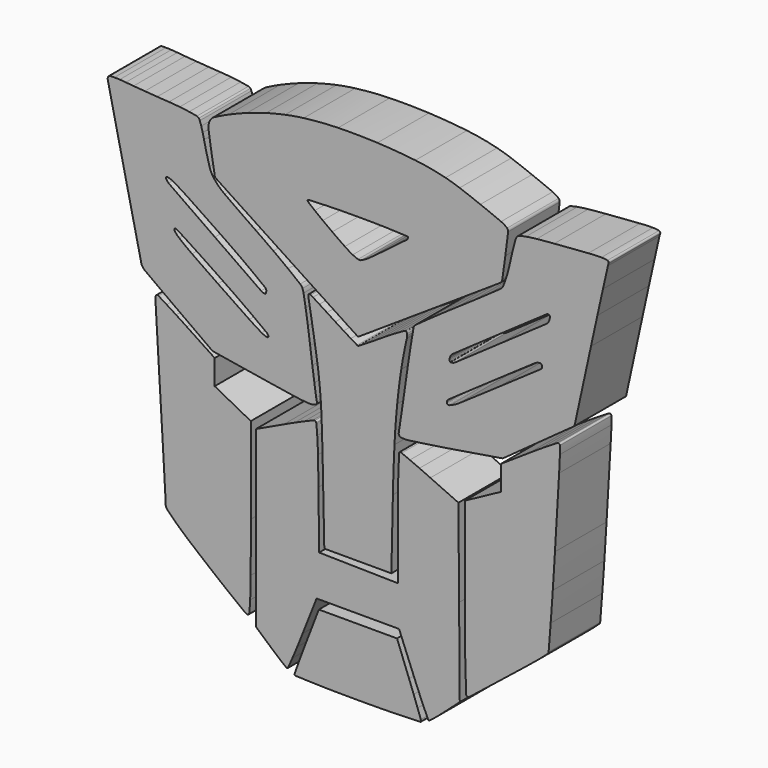
from build123d import *

# Parameters (mm, degrees)
F1_DEPTH = 25


# Not quite as in the source:
# - ends of sketch curves that miss each other by under 0.0002 mm in the source are joined


with BuildPart() as f1:
    # F0 (on Front) → F1 (new body)
    with BuildSketch(Plane.XZ):
        with BuildLine():
            ThreePointArc((-7.7871389968, 96.4009488717), (-14.4802858445, 96.0659455326), (-21.1477259866, 95.3909018942))
            ThreePointArc((-21.1477259866, 95.3909018942), (-24.7777244631, 94.8564824054), (-28.3836838991, 94.1785815164))
            ThreePointArc((-28.3836838991, 94.1785815164), (-32.0904730243, 93.3361025196), (-35.7648669134, 92.3619946955))
            ThreePointArc((-35.7648669134, 92.3619946955), (-39.4624856609, 91.2403059302), (-43.1184530528, 89.9895171458))
            ThreePointArc((-43.1184530528, 89.9895171458), (-46.7206384931, 88.6136238863), (-50.2719786883, 87.1113572979))
            ThreePointArc((-50.2719786883, 87.1113572979), (-53.1174557084, 85.7851246094), (-55.9125031708, 84.3556693195))
            ThreePointArc((-55.9125031708, 84.3556693195), (-56.9599216153, 83.5327385231), (-57.6618821388, 82.4006820555))
            ThreePointArc((-57.6618821388, 82.4006820555), (-58.0273005227, 80.978523326), (-58.0188121091, 79.5101931205))
            ThreePointArc((-58.0188121091, 79.5101931205), (-57.4050586657, 75.2351533659), (-56.7215456466, 70.9707110596))
            Line((-56.7215456466, 70.9707110596), (-55.545967, 64.001086))
            Line((-55.545967, 64.001086), (-30.461838, 47.51707))
            ThreePointArc((-30.461838, 47.51707), (-25.5599805849, 44.2963588564), (-20.6576271192, 41.0764028185))
            ThreePointArc((-20.6576271192, 41.0764028185), (-16.3105522589, 38.2223324949), (-11.9628498638, 35.3692182077))
            ThreePointArc((-11.9628498638, 35.3692182077), (-8.2807722481, 32.9538008658), (-4.5984092513, 30.5388186167))
            ThreePointArc((-4.5984092513, 30.5388186167), (-3.6557973546, 29.9230173812), (-2.7110817564, 29.3104483771))
            Line((-2.7110817564, 29.3104483771), (-0.044454, 27.587842))
            Line((-0.044454, 27.587842), (27.40391, 45.662816))
            ThreePointArc((27.40391, 45.662816), (32.6768790001, 49.136531609), (37.9485342795, 52.6122405762))
            ThreePointArc((37.9485342795, 52.6122405762), (42.4121029737, 55.5583452338), (46.8738502017, 58.5072076951))
            ThreePointArc((46.8738502017, 58.5072076951), (50.8820698473, 61.1582365066), (54.8901678715, 63.8094491942))
            ThreePointArc((54.8901678715, 63.8094491942), (55.0192170204, 63.9027750955), (55.1400437901, 64.0065262248))
            ThreePointArc((55.1400437901, 64.0065262248), (55.6271868144, 64.6463564976), (55.8748182743, 65.4114511053))
            ThreePointArc((55.8748182743, 65.4114511053), (56.4715267421, 69.6147694006), (57.0417758288, 73.8217590227))
            ThreePointArc((57.0417758288, 73.8217590227), (57.596923666, 78.0974834015), (58.1309676384, 82.3758949219))
            ThreePointArc((58.1309676384, 82.3758949219), (58.0590093517, 82.9769076903), (57.7167750279, 83.4761770312))
            ThreePointArc((57.7167750279, 83.4761770312), (56.6161151389, 84.3050714361), (55.392932935, 84.939376844))
            ThreePointArc((55.392932935, 84.939376844), (51.3880107464, 86.5869045709), (47.3681719583, 88.1976948946))
            ThreePointArc((47.3681719583, 88.1976948946), (43.3587549264, 89.7477962193), (39.3261631957, 91.2365685427))
            ThreePointArc((39.3261631957, 91.2365685427), (36.6097303702, 92.1414723377), (33.8522739854, 92.9123759426))
            ThreePointArc((33.8522739854, 92.9123759426), (28.0367501, 94.1819202218), (22.1498009897, 95.0627669114))
            ThreePointArc((22.1498009897, 95.0627669114), (14.802388714, 95.7832710166), (7.4341970002, 96.2451630052))
            ThreePointArc((7.4341970002, 96.2451630052), (-0.1751155832, 96.4554892907), (-7.7871389968, 96.4009488717))
        make_face()
        with BuildLine():
            ThreePointArc((19.0402640372, 68.0878828396), (19.2429014899, 67.9932442976), (19.3193110957, 67.7830539958))
            ThreePointArc((19.3193110957, 67.7830539958), (19.1813400447, 67.2695037039), (18.8389564856, 66.8626336728))
            ThreePointArc((18.8389564856, 66.8626336728), (15.1159629469, 64.0249741693), (11.384749851, 61.1981311973))
            ThreePointArc((11.384749851, 61.1981311973), (7.9259756693, 58.6105934074), (4.4434357694, 56.0551313173))
            ThreePointArc((4.4434357694, 56.0551313173), (2.9054012774, 55.0379035263), (1.2837569665, 54.1600810691))
            ThreePointArc((1.2837569665, 54.1600810691), (0.6198402223, 53.9798990752), (-0.0640028179, 54.0547965969))
            ThreePointArc((-0.0640028179, 54.0547965969), (-1.1212634849, 54.4332391828), (-2.1377660104, 54.9104619803))
            ThreePointArc((-2.1377660104, 54.9104619803), (-3.6865885064, 55.7856963811), (-5.184320766, 56.7457403437))
            ThreePointArc((-5.184320766, 56.7457403437), (-7.6332065318, 58.4369597951), (-10.059751525, 60.1600802708))
            ThreePointArc((-10.059751525, 60.1600802708), (-11.896375827, 61.4957166855), (-13.720253444, 62.8487074074))
            ThreePointArc((-13.720253444, 62.8487074074), (-15.2728438218, 64.0300656839), (-16.8076561206, 65.2344308486))
            ThreePointArc((-16.8076561206, 65.2344308486), (-18.106988474, 66.2756164446), (-19.400562618, 67.3239474687))
            ThreePointArc((-19.400562618, 67.3239474687), (-19.5636563725, 67.5288505749), (-19.6266290148, 67.7830539996))
            ThreePointArc((-19.6266290148, 67.7830539996), (-19.5472806273, 67.9935196361), (-19.3431069986, 68.0878869692))
            ThreePointArc((-19.3431069986, 68.0878869692), (-16.6284187312, 68.2042556562), (-13.9134039882, 68.3127406931))
            ThreePointArc((-13.9134039882, 68.3127406931), (-10.7689410735, 68.4148692664), (-7.6234769951, 68.4791576626))
            ThreePointArc((-7.6234769951, 68.4791576626), (-3.8856986475, 68.5195810383), (-0.147726, 68.5330539999))
            ThreePointArc((-0.147726, 68.5330539999), (3.5898426403, 68.5195815863), (7.327217, 68.4791620031))
            ThreePointArc((7.327217, 68.4791620031), (10.471342585, 68.4148820808), (13.6144659873, 68.3127406712))
            ThreePointArc((13.6144659873, 68.3127406712), (16.3275287109, 68.204261809), (19.0402640372, 68.0878828396))
        make_face(mode=Mode.SUBTRACT)
    extrude(amount=F1_DEPTH)


with BuildPart() as f1b:
    # F0 (on Front) → F1, piece 2 (new body)
    with BuildSketch(Plane.XZ):
        with BuildLine():
            ThreePointArc((-96.2537729873, 85.3507327118), (-96.5128646217, 85.2890918282), (-96.7307979178, 85.1360129205))
            ThreePointArc((-96.7307979178, 85.1360129205), (-97.0917755206, 84.5089297705), (-97.112631726, 83.7856710607))
            ThreePointArc((-97.112631726, 83.7856710607), (-93.8621854047, 69.1270025934), (-90.6031200374, 54.4702479917))
            ThreePointArc((-90.6031200374, 54.4702479917), (-87.3658251329, 39.9600151765), (-84.1164584372, 25.4524809019))
            ThreePointArc((-84.1164584372, 25.4524809019), (-83.7199659075, 24.453163985), (-83.0342755429, 23.6251123838))
            ThreePointArc((-83.0342755429, 23.6251123838), (-82.6998535563, 23.3436135046), (-82.3530924731, 23.077462354))
            ThreePointArc((-82.3530924731, 23.077462354), (-80.4956982376, 21.718412716), (-78.637168479, 20.3609163436))
            ThreePointArc((-78.637168479, 20.3609163436), (-76.4671997257, 18.7807391078), (-74.2939932491, 17.2050176556))
            ThreePointArc((-74.2939932491, 17.2050176556), (-71.8034000507, 15.405667789), (-69.3103408688, 13.6097361823))
            Line((-69.3103408688, 13.6097361823), (-56.472956, 4.375399))
            Line((-56.472956, 4.375399), (-38.495357, 1.454226))
            ThreePointArc((-38.495357, 1.454226), (-31.4405375554, 0.3227131206), (-24.3811449202, -0.7799084822))
            ThreePointArc((-24.3811449202, -0.7799084822), (-21.6792529045, -1.1267782012), (-18.9633119984, -1.3370259701))
            ThreePointArc((-18.9633119984, -1.3370259701), (-17.7740939268, -1.2719497671), (-16.6256430781, -0.9564578015))
            ThreePointArc((-16.6256430781, -0.9564578015), (-16.0801825847, -0.4549294989), (-16.0135623728, 0.2830541794))
            ThreePointArc((-16.0135623728, 0.2830541794), (-16.1696572924, 0.9050190881), (-16.2847309237, 1.5358630114))
            ThreePointArc((-16.2847309237, 1.5358630114), (-16.6410369068, 3.9504441176), (-16.9915906383, 6.3658670521))
            ThreePointArc((-16.9915906383, 6.3658670521), (-17.3966120115, 9.2242411028), (-17.7891888023, 12.0843508916))
            ThreePointArc((-17.7891888023, 12.0843508916), (-18.2195243754, 15.3080541609), (-18.6400329627, 18.5330540048))
            ThreePointArc((-18.6400329627, 18.5330540048), (-19.0673703857, 21.7697354039), (-19.514999314, 25.0036729555))
            ThreePointArc((-19.514999314, 25.0036729555), (-19.9379123744, 27.8992824593), (-20.3859951427, 30.7911039772))
            ThreePointArc((-20.3859951427, 30.7911039772), (-20.7794649567, 33.2167220267), (-21.1862063769, 35.6401499357))
            ThreePointArc((-21.1862063769, 35.6401499357), (-21.3532465447, 36.3773616827), (-21.59848846, 37.0923722183))
            ThreePointArc((-21.59848846, 37.0923722183), (-21.9732756915, 37.7586506091), (-22.504757986, 38.3081220175))
            ThreePointArc((-22.504757986, 38.3081220175), (-24.8446202341, 40.1596416971), (-27.2008603373, 41.9902735619))
            ThreePointArc((-27.2008603373, 41.9902735619), (-30.0334204496, 44.1346996289), (-32.9001829979, 46.2331830029))
            ThreePointArc((-32.9001829979, 46.2331830029), (-36.18789908, 48.5719314894), (-39.5012108958, 50.8742751517))
            ThreePointArc((-39.5012108958, 50.8742751517), (-45.6523102857, 55.1379419489), (-51.7660661609, 59.4549857742))
            ThreePointArc((-51.7660661609, 59.4549857742), (-53.7837081683, 61.1020683225), (-55.5690925953, 62.9984233339))
            ThreePointArc((-55.5690925953, 62.9984233339), (-56.8168721985, 64.8740252319), (-57.6555400889, 66.9648319746))
            ThreePointArc((-57.6555400889, 66.9648319746), (-58.7885511349, 71.1911043774), (-59.7792582331, 75.4529809499))
            ThreePointArc((-59.7792582331, 75.4529809499), (-60.0289354758, 76.5641092849), (-60.2994544999, 77.6703481273))
            ThreePointArc((-60.2994544999, 77.6703481273), (-60.5735343915, 78.6973945218), (-60.8712682044, 79.7178349378))
            ThreePointArc((-60.8712682044, 79.7178349378), (-61.1385492297, 80.5653367753), (-61.422826187, 81.4072899348))
            ThreePointArc((-61.422826187, 81.4072899348), (-61.5894897228, 81.7868130455), (-61.8131691021, 82.1357859227))
            ThreePointArc((-61.8131691021, 82.1357859227), (-62.1442524356, 82.437255471), (-62.5616489036, 82.5993675111))
            ThreePointArc((-62.5616489036, 82.5993675111), (-64.0589330875, 82.868340771), (-65.5606369018, 83.1114296416))
            ThreePointArc((-65.5606369018, 83.1114296416), (-67.3864859195, 83.3659926258), (-69.2184690337, 83.5718196596))
            ThreePointArc((-69.2184690337, 83.5718196596), (-71.306680447, 83.7591826301), (-73.3979489653, 83.9086075563))
            ThreePointArc((-73.3979489653, 83.9086075563), (-75.6759580518, 84.0543797854), (-77.9534739783, 84.2076643151))
            ThreePointArc((-77.9534739783, 84.2076643151), (-80.353219185, 84.376550137), (-82.7524789599, 84.552197537))
            ThreePointArc((-82.7524789599, 84.552197537), (-84.9334852275, 84.7180704744), (-87.1140119613, 84.8901324818))
            ThreePointArc((-87.1140119613, 84.8901324818), (-88.6314119068, 85.0182169847), (-90.1477259837, 85.1585731689))
            ThreePointArc((-90.1477259837, 85.1585731689), (-91.3174272434, 85.2596603406), (-92.4889379873, 85.3370052278))
            ThreePointArc((-92.4889379873, 85.3370052278), (-93.5223197577, 85.3793790407), (-94.5565029997, 85.3911449229))
            ThreePointArc((-94.5565029997, 85.3911449229), (-95.4053438831, 85.3795859207), (-96.2537729873, 85.3507327118))
        make_face()
        with BuildLine():
            ThreePointArc((-59.3567944872, 34.2731742692), (-55.9972836125, 32.023655789), (-52.6471144945, 29.7602482713))
            ThreePointArc((-52.6471144945, 29.7602482713), (-49.2969006577, 27.4672945699), (-45.9649247334, 25.1479183797))
            ThreePointArc((-45.9649247334, 25.1479183797), (-43.09967692, 23.1104822265), (-40.2593773423, 21.0384085368))
            ThreePointArc((-40.2593773423, 21.0384085368), (-37.847218078, 19.247242502), (-35.4436121936, 17.4446147431))
            ThreePointArc((-35.4436121936, 17.4446147431), (-35.0762083676, 17.0688445282), (-34.8370076197, 16.6009001268))
            ThreePointArc((-34.8370076197, 16.6009001268), (-34.9338115917, 16.1374137696), (-35.3847869162, 15.9931523781))
            ThreePointArc((-35.3847869162, 15.9931523781), (-36.434739431, 16.3132384028), (-37.4223486603, 16.7922825805))
            ThreePointArc((-37.4223486603, 16.7922825805), (-39.850939773, 18.2652760205), (-42.2320127336, 19.8139063958))
            ThreePointArc((-42.2320127336, 19.8139063958), (-48.3202958473, 23.922990785), (-54.3977260066, 28.0481099903))
            ThreePointArc((-54.3977260066, 28.0481099903), (-59.4192462656, 31.4891476948), (-64.4192178677, 34.9614221893))
            ThreePointArc((-64.4192178677, 34.9614221893), (-66.9448795818, 36.8007915916), (-69.3975400174, 38.7364319788))
            ThreePointArc((-69.3975400174, 38.7364319788), (-70.3868357697, 39.6671751086), (-71.2419530105, 40.7225249926))
            ThreePointArc((-71.2419530105, 40.7225249926), (-71.2779551583, 41.2555845858), (-70.821382, 41.533054))
            ThreePointArc((-70.821382, 41.533054), (-70.5125688746, 41.4886117713), (-70.2288199075, 41.3588921437))
            ThreePointArc((-70.2288199075, 41.3588921437), (-67.6840559294, 39.718803615), (-65.1418239494, 38.0747930781))
            ThreePointArc((-65.1418239494, 38.0747930781), (-62.2430596459, 36.1834938195), (-59.3567944872, 34.2731742692))
        make_face(mode=Mode.SUBTRACT)
        with BuildLine():
            ThreePointArc((-65.9710112801, 53.7295375814), (-59.7586832447, 49.5574335995), (-53.5607942831, 45.3639095831))
            ThreePointArc((-53.5607942831, 45.3639095831), (-50.116226478, 43.0005705594), (-46.6943279492, 40.6045260717))
            ThreePointArc((-46.6943279492, 40.6045260717), (-43.7861024137, 38.5144080861), (-40.9096902696, 36.3807206423))
            ThreePointArc((-40.9096902696, 36.3807206423), (-38.4722911887, 34.533695248), (-36.0449389935, 32.6734860084))
            ThreePointArc((-36.0449389935, 32.6734860084), (-35.7524022942, 32.3158838689), (-35.647726, 31.865884))
            ThreePointArc((-35.647726, 31.865884), (-35.6540905892, 31.6101878361), (-35.6731689905, 31.3551249991))
            ThreePointArc((-35.6731689905, 31.3551249991), (-35.7035169552, 31.1383121393), (-35.7508917516, 30.9245729346))
            ThreePointArc((-35.7508917516, 30.9245729346), (-35.7998305298, 30.7689599306), (-35.8631747683, 30.6186338892))
            ThreePointArc((-35.8631747683, 30.6186338892), (-35.9186911066, 30.5562343197), (-35.998931, 30.533054))
            ThreePointArc((-35.998931, 30.533054), (-36.8646507225, 30.665724365), (-37.6509101006, 31.0515588556))
            ThreePointArc((-37.6509101006, 31.0515588556), (-46.6192802409, 37.3031499852), (-55.5814697672, 43.5635983329))
            ThreePointArc((-55.5814697672, 43.5635983329), (-64.5578975876, 49.8468061519), (-73.5284907469, 56.1383413606))
            ThreePointArc((-73.5284907469, 56.1383413606), (-74.1124708559, 56.7115802195), (-74.4806178517, 57.4424040463))
            ThreePointArc((-74.4806178517, 57.4424040463), (-74.3587456166, 57.9635705409), (-73.843835953, 58.1096371795))
            ThreePointArc((-73.843835953, 58.1096371795), (-72.5830248753, 57.6878334918), (-71.3897787884, 57.1015513666))
            ThreePointArc((-71.3897787884, 57.1015513666), (-68.652548501, 55.4602933542), (-65.9710112801, 53.7295375814))
        make_face(mode=Mode.SUBTRACT)
    extrude(amount=F1_DEPTH)


with BuildPart() as f1c:
    # F0 (on Front) → F1, piece 3 (new body)
    with BuildSketch(Plane.XZ):
        with BuildLine():
            ThreePointArc((89.2154619727, 85.1472903689), (82.6198071673, 84.6495571544), (76.0255429705, 84.1337273711))
            ThreePointArc((76.0255429705, 84.1337273711), (72.6101720334, 83.8451359582), (69.1977680446, 83.5233555502))
            ThreePointArc((69.1977680446, 83.5233555502), (67.1055980703, 83.2750485385), (65.0245370305, 82.9463898282))
            ThreePointArc((65.0245370305, 82.9463898282), (63.6907525773, 82.6722710823), (62.373575997, 82.3270640104))
            ThreePointArc((62.373575997, 82.3270640104), (61.8030345075, 82.0287946116), (61.3922747431, 81.5330541382))
            ThreePointArc((61.3922747431, 81.5330541382), (61.1645324131, 81.0489311988), (60.9899338434, 80.5432070448))
            ThreePointArc((60.9899338434, 80.5432070448), (60.641980812, 79.3029240012), (60.3071512576, 78.0590339321))
            ThreePointArc((60.3071512576, 78.0590339321), (59.9245847977, 76.5672438379), (59.5618207653, 75.0705150552))
            ThreePointArc((59.5618207653, 75.0705150552), (59.1878409128, 73.4436528487), (58.8308197635, 71.8129850505))
            ThreePointArc((58.8308197635, 71.8129850505), (58.4586883075, 70.182547326), (58.0408514653, 68.5632198729))
            ThreePointArc((58.0408514653, 68.5632198729), (57.6054100726, 67.0721205742), (57.1179392093, 65.5972109267))
            ThreePointArc((57.1179392093, 65.5972109267), (56.673004376, 64.3883546824), (56.1897932506, 63.1942828939))
            ThreePointArc((56.1897932506, 63.1942828939), (55.8841216606, 62.6535633799), (55.46408825, 62.1959777116))
            ThreePointArc((55.46408825, 62.1959777116), (54.8854306009, 61.7191814499), (54.2837419005, 61.271800141))
            ThreePointArc((54.2837419005, 61.271800141), (51.9886827088, 59.6557489947), (49.6905958734, 58.0440061809))
            ThreePointArc((49.6905958734, 58.0440061809), (46.9662500392, 56.1439789773), (44.2354900032, 54.2531819953))
            ThreePointArc((44.2354900032, 54.2531819953), (41.1567823399, 52.1345582044), (38.0730451522, 50.0232617771))
            ThreePointArc((38.0730451522, 50.0232617771), (35.0241609229, 47.9315647513), (31.9842612033, 45.8268317077))
            ThreePointArc((31.9842612033, 45.8268317077), (29.3672149298, 43.9936970177), (26.762354013, 42.1432879818))
            ThreePointArc((26.762354013, 42.1432879818), (24.5167023314, 40.5332207907), (22.2744954416, 38.9183597736))
            ThreePointArc((22.2744954416, 38.9183597736), (21.9716305662, 38.6509910872), (21.7266319607, 38.3297610243))
            ThreePointArc((21.7266319607, 38.3297610243), (21.5498642471, 37.9711086197), (21.4445107737, 37.5853898664))
            ThreePointArc((21.4445107737, 37.5853898664), (21.0329089052, 35.1827734341), (20.6276378585, 32.7790810237))
            ThreePointArc((20.6276378585, 32.7790810237), (20.1706376553, 29.9837972058), (19.734105083, 27.1852439874))
            ThreePointArc((19.734105083, 27.1852439874), (19.2502433865, 23.9550344485), (18.7818475055, 20.7225460705))
            ThreePointArc((18.7818475055, 20.7225460705), (18.3102060171, 17.425863698), (17.8346615468, 14.1297420657))
            ThreePointArc((17.8346615468, 14.1297420657), (17.3974323323, 11.1284167998), (16.9555030645, 8.1277799904))
            ThreePointArc((16.9555030645, 8.1277799904), (16.5815878424, 5.6123852174), (16.2048608534, 3.097410022))
            ThreePointArc((16.2048608534, 3.097410022), (16.061082094, 2.189064885), (15.9032614467, 1.2830539186))
            ThreePointArc((15.9032614467, 1.2830539186), (15.783162503, 0.5022628604), (15.7062931254, -0.2839620088))
            ThreePointArc((15.7062931254, -0.2839620088), (15.7520579398, -0.6680309145), (15.9359828698, -1.0082881061))
            ThreePointArc((15.9359828698, -1.0082881061), (16.2299154377, -1.2521503326), (16.5943069953, -1.366535043))
            ThreePointArc((16.5943069953, -1.366535043), (17.3596370565, -1.4282185637), (18.1272740018, -1.4446042211))
            ThreePointArc((18.1272740018, -1.4446042211), (19.0352481457, -1.4087441848), (19.9392050733, -1.3161975467))
            ThreePointArc((19.9392050733, -1.3161975467), (22.5804663646, -0.9566792318), (25.2202789469, -0.5866736265))
            ThreePointArc((25.2202789469, -0.5866736265), (28.3660344562, -0.1300398614), (31.5090790244, 0.3448948414))
            ThreePointArc((31.5090790244, 0.3448948414), (34.97926572, 0.8872746037), (38.447078053, 1.4446336748))
            Line((38.447078053, 1.4446336748), (56.041883, 4.31153))
            Line((56.041883, 4.31153), (69.947078, 14.352186))
            Line((69.947078, 14.352186), (83.852274, 24.392843))
            Line((83.852274, 24.392843), (90.252589, 53.712948))
            ThreePointArc((90.252589, 53.712948), (91.4925357583, 59.3779849826), (92.7388156256, 65.0416320826))
            ThreePointArc((92.7388156256, 65.0416320826), (93.8186280965, 69.9154935845), (94.9069585237, 74.7874601068))
            ThreePointArc((94.9069585237, 74.7874601068), (95.8623993828, 79.0425370385), (96.8197624813, 83.2971818916))
            ThreePointArc((96.8197624813, 83.2971818916), (96.948802538, 83.7947825452), (97.1095786237, 84.2830537721))
            ThreePointArc((97.1095786237, 84.2830537721), (97.06920051, 84.802039619), (96.650832937, 85.1117897034))
            ThreePointArc((96.650832937, 85.1117897034), (95.4713848631, 85.2964177028), (94.2788939987, 85.3525501877))
            ThreePointArc((94.2788939987, 85.3525501877), (91.7454622412, 85.2922449893), (89.2154619727, 85.1472903689))
        make_face()
        with BuildLine():
            ThreePointArc((71.2901080779, 40.9478240276), (71.3366194817, 40.7697058821), (71.352274, 40.586282))
            ThreePointArc((71.352274, 40.586282), (71.2152992095, 40.0283989811), (70.8355259701, 39.597391043))
            ThreePointArc((70.8355259701, 39.597391043), (62.6973121238, 33.941759756), (54.5544069388, 28.2928850884))
            ThreePointArc((54.5544069388, 28.2928850884), (46.8760074226, 22.9868159543), (39.1828339128, 17.7021901273))
            ThreePointArc((39.1828339128, 17.7021901273), (37.4465426711, 16.6529789869), (35.6022742163, 15.8078604469))
            ThreePointArc((35.6022742163, 15.8078604469), (35.3674798889, 15.7360499106), (35.124524015, 15.7005877828))
            ThreePointArc((35.124524015, 15.7005877828), (34.9173708214, 15.7121201099), (34.7194621074, 15.7743902346))
            ThreePointArc((34.7194621074, 15.7743902346), (34.5671586584, 15.8745054107), (34.4518296637, 16.0156388016))
            ThreePointArc((34.4518296637, 16.0156388016), (34.3776103338, 16.1912941169), (34.352274, 16.380295))
            ThreePointArc((34.352274, 16.380295), (34.5193482422, 17.062291314), (34.9827350319, 17.5898379544))
            ThreePointArc((34.9827350319, 17.5898379544), (43.4213344835, 23.4781108114), (51.8666885709, 29.3566916173))
            ThreePointArc((51.8666885709, 29.3566916173), (60.2045000943, 35.1431630477), (68.5517898917, 40.9159531568))
            ThreePointArc((68.5517898917, 40.9159531568), (69.4948618687, 41.37520419), (70.531867, 41.533054))
            ThreePointArc((70.531867, 41.533054), (70.6925084296, 41.5146363017), (70.8448130166, 41.4603390339))
            ThreePointArc((70.8448130166, 41.4603390339), (70.9883549067, 41.3710127332), (71.1112795853, 41.2549396407))
            ThreePointArc((71.1112795853, 41.2549396407), (71.2150728044, 41.1097545148), (71.2901080779, 40.9478240276))
        make_face(mode=Mode.SUBTRACT)
        with BuildLine():
            ThreePointArc((74.2346608798, 57.7667500306), (74.1520882452, 57.4782338012), (74.0528048941, 57.1950330407))
            ThreePointArc((74.0528048941, 57.1950330407), (73.5749472999, 56.3500031791), (72.8710412628, 55.6814676251))
            ThreePointArc((72.8710412628, 55.6814676251), (64.0711456062, 49.5210206721), (55.2636919106, 43.3713841282))
            ThreePointArc((55.2636919106, 43.3713841282), (46.4420198884, 37.2277711589), (37.6129576322, 31.0947835301))
            ThreePointArc((37.6129576322, 31.0947835301), (36.7582813905, 30.6767653692), (35.817772, 30.533054))
            ThreePointArc((35.817772, 30.533054), (35.6988540782, 30.5634856395), (35.6091719688, 30.6472989801))
            ThreePointArc((35.6091719688, 30.6472989801), (35.5295940876, 30.8022168743), (35.4804206434, 30.9692921251))
            ThreePointArc((35.4804206434, 30.9692921251), (35.4496090728, 31.2081942088), (35.449461259, 31.4490749836))
            ThreePointArc((35.449461259, 31.4490749836), (35.4784478337, 31.7350992266), (35.5289498139, 32.0181180405))
            ThreePointArc((35.5289498139, 32.0181180405), (35.9196279277, 32.940707501), (36.6192008731, 33.657923181))
            ThreePointArc((36.6192008731, 33.657923181), (45.6637493558, 39.9911357598), (54.7181795756, 46.3102126092))
            ThreePointArc((54.7181795756, 46.3102126092), (63.8945086886, 52.6962651947), (73.0777928608, 59.0723122007))
            ThreePointArc((73.0777928608, 59.0723122007), (73.6683708491, 59.2312585329), (74.2258130486, 58.9796550504))
            ThreePointArc((74.2258130486, 58.9796550504), (74.3015573716, 58.87369664), (74.3344269911, 58.7476649994))
            ThreePointArc((74.3344269911, 58.7476649994), (74.3410716505, 58.527109382), (74.3290760571, 58.3067799945))
            ThreePointArc((74.3290760571, 58.3067799945), (74.2921938377, 58.0349597905), (74.2346608798, 57.7667500306))
        make_face(mode=Mode.SUBTRACT)
    extrude(amount=F1_DEPTH)


with BuildPart() as f1d:
    # F0 (on Front) → F1, piece 4 (new body)
    with BuildSketch(Plane.XZ):
        with BuildLine():
            ThreePointArc((-19.312651238, 35.1537330751), (-19.235162014, 34.491616874), (-19.1335902241, 33.8327651341))
            ThreePointArc((-19.1335902241, 33.8327651341), (-17.6669798117, 25.1600642614), (-16.2640300828, 16.4768379869))
            ThreePointArc((-16.2640300828, 16.4768379869), (-15.5086983548, 11.1784218965), (-14.9117196327, 5.8598360357))
            ThreePointArc((-14.9117196327, 5.8598360357), (-14.4778240215, 0.5625488662), (-14.2044595977, -4.7454440217))
            ThreePointArc((-14.2044595977, -4.7454440217), (-13.9248788775, -13.3552445475), (-13.7117391558, -21.9669460033))
            Line((-13.7117391558, -21.9669460033), (-13.147726, -48.966946))
            Line((-13.147726, -48.966946), (-0.147726, -48.966946))
            Line((-0.147726, -48.966946), (12.852274, -48.966946))
            Line((12.852274, -48.966946), (13.448144, -21.966946))
            ThreePointArc((13.448144, -21.966946), (13.6984754067, -13.3136884498), (14.0674139302, -4.6646759965))
            ThreePointArc((14.0674139302, -4.6646759965), (14.5072910177, 2.4684348786), (15.1196920966, 9.5888089905))
            ThreePointArc((15.1196920966, 9.5888089905), (15.8151751521, 15.7640732074), (16.6863968648, 21.9170040211))
            ThreePointArc((16.6863968648, 21.9170040211), (17.6801772765, 27.6193191923), (18.8743745449, 33.283053875))
            ThreePointArc((18.8743745449, 33.283053875), (18.9547478781, 33.7115605156), (19.0005986907, 34.1451219548))
            ThreePointArc((19.0005986907, 34.1451219548), (18.9997620047, 34.5103435918), (18.9496868706, 34.8721169731))
            ThreePointArc((18.9496868706, 34.8721169731), (18.869781835, 35.1254792841), (18.7409779969, 35.3578299979))
            ThreePointArc((18.7409779969, 35.3578299979), (18.5951071109, 35.4866002357), (18.406157, 35.533054))
            ThreePointArc((18.406157, 35.533054), (18.0651523944, 35.4893783042), (17.7461621161, 35.3611717923))
            ThreePointArc((17.7461621161, 35.3611717923), (16.4737234864, 34.6439996741), (15.2066281338, 33.9174287687))
            ThreePointArc((15.2066281338, 33.9174287687), (13.7141375875, 33.0397631446), (12.2345221828, 32.1405617041))
            ThreePointArc((12.2345221828, 32.1405617041), (10.5602180005, 31.0949877443), (8.8962424571, 30.0330532915))
            ThreePointArc((8.8962424571, 30.0330532915), (7.2476129796, 28.9750328068), (5.5939897954, 27.9248343239))
            ThreePointArc((5.5939897954, 27.9248343239), (4.1681254921, 27.0314313749), (2.7356430167, 26.1486789726))
            ThreePointArc((2.7356430167, 26.1486789726), (1.4862621967, 25.3869196879), (0.2353282432, 24.6277135984))
            ThreePointArc((0.2353282432, 24.6277135984), (0.0722674291, 24.5571629559), (-0.103758, 24.533054))
            ThreePointArc((-0.103758, 24.533054), (-0.2794913204, 24.5569730537), (-0.4424390212, 24.6269899647))
            ThreePointArc((-0.4424390212, 24.6269899647), (-1.6582118246, 25.3593834048), (-2.8724058625, 26.0943912267))
            ThreePointArc((-2.8724058625, 26.0943912267), (-4.2659789807, 26.9473300393), (-5.6529981954, 27.8108856889))
            ThreePointArc((-5.6529981954, 27.8108856889), (-7.2604241124, 28.8256614736), (-8.862895186, 29.8482437101))
            ThreePointArc((-8.862895186, 29.8482437101), (-10.494132104, 30.8937226201), (-12.1263240469, 31.9377099267))
            ThreePointArc((-12.1263240469, 31.9377099267), (-13.6009897876, 32.8787009422), (-15.0768211344, 33.8178627885))
            ThreePointArc((-15.0768211344, 33.8178627885), (-16.3169662191, 34.605246137), (-17.5577581241, 35.3916098041))
            ThreePointArc((-17.5577581241, 35.3916098041), (-17.968447938, 35.647658044), (-18.3826680562, 35.8979549055))
            ThreePointArc((-18.3826680562, 35.8979549055), (-18.6372850004, 36.0075377315), (-18.9115280026, 36.0478978362))
            ThreePointArc((-18.9115280026, 36.0478978362), (-19.1042846855, 35.9896340436), (-19.2274696797, 35.8303378835))
            ThreePointArc((-19.2274696797, 35.8303378835), (-19.3080270675, 35.4968152884), (-19.312651238, 35.1537330751))
        make_face()
    extrude(amount=F1_DEPTH)


with BuildPart() as f1e:
    # F0 (on Front) → F1, piece 5 (new body)
    with BuildSketch(Plane.XZ):
        with BuildLine():
            ThreePointArc((-78.5877622663, 15.7612490563), (-78.6246305869, 15.523451953), (-78.635380369, 15.2830539964))
            ThreePointArc((-78.635380369, 15.2830539964), (-78.624694272, 14.7950041505), (-78.6022842651, 14.3073519846))
            ThreePointArc((-78.6022842651, 14.3073519846), (-78.3235370403, 9.5069047043), (-78.0441949137, 4.706492005))
            ThreePointArc((-78.0441949137, 4.706492005), (-77.7241897293, -0.7604282356), (-77.4011334834, -6.2271690287))
            ThreePointArc((-77.4011334834, -6.2271690287), (-77.0217797901, -12.5971248642), (-76.6401713197, -18.9669460192))
            ThreePointArc((-76.6401713197, -18.9669460192), (-76.2579351721, -25.3634903314), (-75.8798952797, -31.7602840164))
            ThreePointArc((-75.8798952797, -31.7602840164), (-75.5563489567, -37.3132193006), (-75.2383670579, -42.8664760033))
            ThreePointArc((-75.2383670579, -42.8664760033), (-74.9668656908, -47.6645229416), (-74.6970149631, -52.4626629979))
            ThreePointArc((-74.6970149631, -52.4626629979), (-74.6645478452, -53.2243436403), (-74.6525169918, -53.986621))
            ThreePointArc((-74.6525169918, -53.986621), (-74.5053157086, -54.7482969959), (-74.0880080733, -55.4022640692))
            ThreePointArc((-74.0880080733, -55.4022640692), (-72.5731480828, -56.9648255889), (-71.0169967098, -58.4862696951))
            ThreePointArc((-71.0169967098, -58.4862696951), (-68.7609744179, -60.5743282153), (-66.4474588733, -62.5984998511))
            ThreePointArc((-66.4474588733, -62.5984998511), (-63.0621782633, -65.4495248347), (-59.649267117, -68.2674151432))
            ThreePointArc((-59.649267117, -68.2674151432), (-56.7269178477, -70.6446095768), (-53.7930690069, -73.0075970086))
            ThreePointArc((-53.7930690069, -73.0075970086), (-51.2116677049, -75.0611747748), (-48.6155271982, -77.0960872548))
            ThreePointArc((-48.6155271982, -77.0960872548), (-46.3930265662, -78.819509258), (-44.1650019894, -80.5357839862))
            ThreePointArc((-44.1650019894, -80.5357839862), (-43.677677655, -80.8569316562), (-43.1492669739, -81.1047279321))
            ThreePointArc((-43.1492669739, -81.1047279321), (-42.5796968724, -81.0531155876), (-42.2725871252, -80.5706660967))
            ThreePointArc((-42.2725871252, -80.5706660967), (-42.0505800799, -78.2150390508), (-41.9046358984, -75.853478959))
            ThreePointArc((-41.9046358984, -75.853478959), (-41.7550238718, -71.6235416218), (-41.6920984973, -67.3914270023))
            ThreePointArc((-41.6920984973, -67.3914270023), (-41.6588185849, -57.7946406476), (-41.647726, -48.197803))
            Line((-41.647726, -48.197803), (-41.647726, -14.714682))
            Line((-41.647726, -14.714682), (-48.647726, -11.036286))
            Line((-48.647726, -11.036286), (-55.647726, -7.35789))
            Line((-55.647726, -7.35789), (-55.647726, -2.549037))
            Line((-55.647726, -2.549037), (-55.647726, 2.259816))
            Line((-55.647726, 2.259816), (-66.441105, 9.396435))
            ThreePointArc((-66.441105, 9.396435), (-68.531290449, 10.7700346509), (-70.6291760377, 12.1318449416))
            ThreePointArc((-70.6291760377, 12.1318449416), (-72.4452835756, 13.2922444352), (-74.27149791, 14.436672145))
            ThreePointArc((-74.27149791, 14.436672145), (-75.8556785064, 15.4167430614), (-77.4425658874, 16.3924251837))
            ThreePointArc((-77.4425658874, 16.3924251837), (-77.6821080881, 16.4972238552), (-77.941105, 16.533054))
            ThreePointArc((-77.941105, 16.533054), (-78.0837136151, 16.5083760268), (-78.2097370925, 16.4372121132))
            ThreePointArc((-78.2097370925, 16.4372121132), (-78.3360063826, 16.3122986235), (-78.4365291998, 16.165866111))
            ThreePointArc((-78.4365291998, 16.165866111), (-78.5272771674, 15.9692132363), (-78.5877622663, 15.7612490563))
        make_face()
    extrude(amount=F1_DEPTH)


with BuildPart() as f1f:
    # F0 (on Front) → F1, piece 6 (new body)
    with BuildSketch(Plane.XZ):
        with BuildLine():
            ThreePointArc((70.2767649437, 12.1198830871), (68.1854541091, 10.7577452915), (66.1022739448, 9.3832050831))
            Line((66.1022739448, 9.3832050831), (55.352274, 2.244105))
            Line((55.352274, 2.244105), (55.352274, -2.540996))
            Line((55.352274, -2.540996), (55.352274, -7.326097))
            Line((55.352274, -7.326097), (48.352274, -11.106957))
            Line((48.352274, -11.106957), (41.352274, -14.887817))
            Line((41.352274, -14.887817), (41.352274, -48.177381))
            ThreePointArc((41.352274, -48.177381), (41.3672499045, -55.3176903031), (41.4121720027, -62.457874))
            ThreePointArc((41.4121720027, -62.457874), (41.4832868808, -67.6374054417), (41.6097137595, -72.8158820072))
            ThreePointArc((41.6097137595, -72.8158820072), (41.7379326469, -76.9175496643), (41.8784629457, -81.0188139662))
            ThreePointArc((41.8784629457, -81.0188139662), (42.0202120384, -81.3366472968), (42.342909, -81.466946))
            ThreePointArc((42.342909, -81.466946), (42.8531873861, -81.3804313817), (43.3064330623, -81.1305570784))
            ThreePointArc((43.3064330623, -81.1305570784), (49.9918074406, -75.8111439859), (56.6738611331, -70.487560167))
            ThreePointArc((56.6738611331, -70.487560167), (62.6780548591, -65.6823990578), (68.6640618448, -60.8546008083))
            ThreePointArc((68.6640618448, -60.8546008083), (71.136517142, -58.7751198642), (73.5295199968, -56.6046789966))
            ThreePointArc((73.5295199968, -56.6046789966), (73.7363566309, -56.3217811607), (73.8274935217, -55.9833929621))
            ThreePointArc((73.8274935217, -55.9833929621), (74.2252225771, -50.9283882677), (74.6184319114, -45.8730299932))
            ThreePointArc((74.6184319114, -45.8730299932), (75.044868733, -40.15324442), (75.4397254957, -34.4311920328))
            ThreePointArc((75.4397254957, -34.4311920328), (75.874047342, -27.6997895564), (76.2854263056, -20.9669460182))
            ThreePointArc((76.2854263056, -20.9669460182), (77.0960695341, -7.2783871163), (77.9020861446, 6.4104449915))
            ThreePointArc((77.9020861446, 6.4104449915), (78.0718708018, 9.6255518127), (78.2038093944, 12.8424339861))
            ThreePointArc((78.2038093944, 12.8424339861), (78.2300192494, 14.3997757577), (78.1992947966, 15.9570349923))
            ThreePointArc((78.1992947966, 15.9570349923), (78.0163995331, 16.3633161654), (77.6022740017, 16.527678768))
            ThreePointArc((77.6022740017, 16.527678768), (77.3287894411, 16.4883532575), (77.0758461556, 16.377177746))
            ThreePointArc((77.0758461556, 16.377177746), (75.493811166, 15.4044041978), (73.9147740535, 14.4267719139))
            ThreePointArc((73.9147740535, 14.4267719139), (72.0904533868, 13.2817111144), (70.2767649437, 12.1198830871))
        make_face()
    extrude(amount=F1_DEPTH)


with BuildPart() as f1g:
    # F0 (on Front) → F1, piece 7 (new body)
    with BuildSketch(Plane.XZ):
        with BuildLine():
            ThreePointArc((-24.6895030525, -9.7298568846), (-26.7971667476, -10.6978058187), (-28.8977260507, -11.6810768927))
            Line((-28.8977260507, -11.6810768927), (-39.647726, -16.760938))
            Line((-39.647726, -16.760938), (-39.647726, -50.531103))
            Line((-39.647726, -50.531103), (-39.647726, -84.301268))
            Line((-39.647726, -84.301268), (-33.897726, -89.369962))
            ThreePointArc((-33.897726, -89.369962), (-32.7791509732, -90.3469126516), (-31.6516549322, -91.3135539202))
            ThreePointArc((-31.6516549322, -91.3135539202), (-30.6639232355, -92.1406846003), (-29.6646892441, -92.9538823043))
            ThreePointArc((-29.6646892441, -92.9538823043), (-28.8082759525, -93.636736905), (-27.9478041362, -94.314470174))
            ThreePointArc((-27.9478041362, -94.314470174), (-27.765991552, -94.4147795403), (-27.5618540046, -94.4528011918))
            ThreePointArc((-27.5618540046, -94.4528011918), (-27.3709993237, -94.3999279004), (-27.241644379, -94.2499668319))
            ThreePointArc((-27.241644379, -94.2499668319), (-26.3970185144, -92.3380113617), (-25.557681445, -90.4237282424))
            ThreePointArc((-25.557681445, -90.4237282424), (-24.6061090145, -88.2110237628), (-23.6797903692, -85.9876288487))
            ThreePointArc((-23.6797903692, -85.9876288487), (-22.6116323914, -83.3559801909), (-21.5618538281, -80.7169460677))
            Line((-21.5618538281, -80.7169460677), (-16.147726, -66.966946))
            Line((-16.147726, -66.966946), (-0.147726, -66.966946))
            Line((-0.147726, -66.966946), (15.852274, -66.966946))
            Line((15.852274, -66.966946), (21.352274, -80.702874))
            ThreePointArc((21.352274, -80.702874), (22.4179925963, -83.3399501689), (23.500566241, -85.9701518999))
            ThreePointArc((23.500566241, -85.9701518999), (24.4378679409, -88.1940301928), (25.3983230876, -90.4080074015))
            ThreePointArc((25.3983230876, -90.4080074015), (26.2470198349, -92.330543637), (27.1002816082, -94.2510581747))
            ThreePointArc((27.1002816082, -94.2510581747), (27.2222904272, -94.3956841113), (27.4026570061, -94.4528737605))
            ThreePointArc((27.4026570061, -94.4528737605), (27.5954188917, -94.4240828925), (27.7668400083, -94.3313420105))
            ThreePointArc((27.7668400083, -94.3313420105), (28.6201060885, -93.651696349), (29.4694517538, -92.9671576963))
            ThreePointArc((29.4694517538, -92.9671576963), (30.458749, -92.153435133), (31.4364137453, -91.3257727034))
            ThreePointArc((31.4364137453, -91.3257727034), (32.5555301178, -90.3556897691), (33.6656766291, -89.3753545838))
            Line((33.6656766291, -89.3753545838), (39.378314, -84.283764))
            Line((39.378314, -84.283764), (39.115294, -50.341327))
            Line((39.115294, -50.341327), (38.852274, -16.398889))
            Line((38.852274, -16.398889), (27.977811, -11.432918))
            ThreePointArc((27.977811, -11.432918), (25.8651077278, -10.4753604967), (23.7470032156, -9.5298105133))
            ThreePointArc((23.7470032156, -9.5298105133), (21.8972094529, -8.7198036551), (20.0405328355, -7.9257003891))
            ThreePointArc((20.0405328355, -7.9257003891), (18.447565958, -7.2557060334), (16.852286146, -6.5912376478))
            ThreePointArc((16.852286146, -6.5912376478), (16.5461730445, -6.4983207014), (16.227811, -6.466946))
            ThreePointArc((16.227811, -6.466946), (15.9816591218, -6.5656935422), (15.8719976442, -6.8071809841))
            ThreePointArc((15.8719976442, -6.8071809841), (15.7360960262, -9.9453826571), (15.6094639375, -13.0839720364))
            ThreePointArc((15.6094639375, -13.0839720364), (15.4902630505, -16.7191374273), (15.4152005894, -20.3554820086))
            ThreePointArc((15.4152005894, -20.3554820086), (15.3680037734, -24.6741223803), (15.3522740002, -28.992992))
            Line((15.3522740002, -28.992992), (15.352274, -51.519038))
            Line((15.352274, -51.519038), (0.102274, -51.242992))
            Line((0.102274, -51.242992), (-15.147726, -50.966946))
            Line((-15.147726, -50.966946), (-15.416858, -28.716946))
            ThreePointArc((-15.416858, -28.716946), (-15.4972594865, -23.2158170681), (-15.6053742307, -17.7151630051))
            ThreePointArc((-15.6053742307, -17.7151630051), (-15.7131406713, -14.5001832099), (-15.8937673544, -11.2884729563))
            ThreePointArc((-15.8937673544, -11.2884729563), (-16.0574146538, -9.1866607687), (-16.2638405151, -7.088618056))
            ThreePointArc((-16.2638405151, -7.088618056), (-16.4798430547, -6.6812185127), (-16.9168580408, -6.5340802519))
            ThreePointArc((-16.9168580408, -6.5340802519), (-17.3457751948, -6.5943081234), (-17.7583160013, -6.7262449969))
            ThreePointArc((-17.7583160013, -6.7262449969), (-19.3530321053, -7.3955099733), (-20.9439711429, -8.0737046674))
            ThreePointArc((-20.9439711429, -8.0737046674), (-22.8211091149, -8.8918930812), (-24.6895030525, -9.7298568846))
        make_face()
    extrude(amount=F1_DEPTH)


with BuildPart() as f1h:
    # F0 (on Front) → F1, piece 8 (new body)
    with BuildSketch(Plane.XZ):
        with BuildLine():
            Line((-15.26552, -70.466946), (-19.973029, -82.716946))
            ThreePointArc((-19.973029, -82.716946), (-20.8793685622, -85.0897696933), (-21.7760952724, -87.4662428979))
            ThreePointArc((-21.7760952724, -87.4662428979), (-22.5409224704, -89.5251658954), (-23.2928877498, -91.5888210903))
            ThreePointArc((-23.2928877498, -91.5888210903), (-23.9356619381, -93.3757689512), (-24.5747961615, -95.1640219425))
            ThreePointArc((-24.5747961615, -95.1640219425), (-24.6446995809, -95.4364066819), (-24.6641321137, -95.7169460025))
            ThreePointArc((-24.6641321137, -95.7169460025), (-24.5739709508, -95.9298763833), (-24.362172985, -96.0226665633))
            ThreePointArc((-24.362172985, -96.0226665633), (-20.909024206, -96.1378171735), (-17.4556700166, -96.2466335418))
            ThreePointArc((-17.4556700166, -96.2466335418), (-13.4998864682, -96.348735804), (-9.5433080014, -96.4130411242))
            ThreePointArc((-9.5433080014, -96.4130411242), (-4.8455943267, -96.4534714649), (-0.147726, -96.4669459998))
            ThreePointArc((-0.147726, -96.4669459998), (4.5501013253, -96.4534718464), (9.247774, -96.4130420036))
            ThreePointArc((9.247774, -96.4130420036), (13.2042169686, -96.3487355642), (17.1598650011, -96.2466330364))
            ThreePointArc((17.1598650011, -96.2466330364), (20.6130367017, -96.1378168743), (24.066003014, -96.0226674092))
            ThreePointArc((24.066003014, -96.0226674092), (24.2776298, -95.9298501335), (24.3674778687, -95.7169459973))
            ThreePointArc((24.3674778687, -95.7169459973), (24.3479087935, -95.4363634044), (24.27847633, -95.1638038835))
            ThreePointArc((24.27847633, -95.1638038835), (23.6452559389, -93.3756721673), (23.0084316466, -91.5888207688))
            ThreePointArc((23.0084316466, -91.5888207688), (22.2634358701, -89.5252099968), (21.5057141612, -87.4662379401))
            ThreePointArc((21.5057141612, -87.4662379401), (20.6174032584, -85.0898043803), (19.7195852192, -82.7169462972))
            Line((19.7195852192, -82.7169462972), (15.05649, -70.466946))
            Line((15.05649, -70.466946), (-0.104515, -70.466946))
            Line((-0.104515, -70.466946), (-15.26552, -70.466946))
        make_face()
    extrude(amount=F1_DEPTH)


solid = Compound([f1.part, f1b.part, f1c.part, f1d.part, f1e.part, f1f.part, f1g.part, f1h.part])
